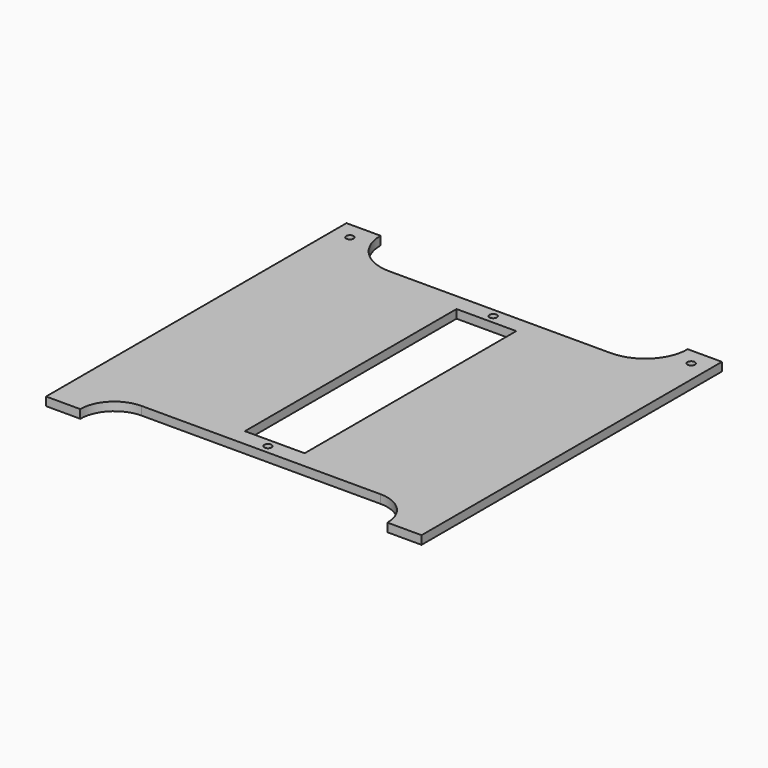
from build123d import *

# Parameters (mm, degrees)
F1_DEPTH = 5
F2_W     = 35
F2_H     = 155
F3_DEPTH = 5.001
F4_R     = 2.15
F5_DEPTH = 5.001


# Not quite as in the source:
# - a feature names something its author has since deleted; it is built from what else it names


with BuildPart() as f1:
    # F0 (on Top) → F1 (new body)
    with BuildSketch(Plane.XY):
        with BuildLine():
            Line((-39.5881515363, 113.7799814343), (-59.5881515363, 113.7799814343))
            Line((-59.5881515363, 113.7799814343), (-59.5881515363, -106.2200185657))
            Line((-59.5881515363, -106.2200185657), (-39.5881515363, -106.2200185657))
            ThreePointArc((-39.5881515363, -106.2200185657), (-33.7302871601, -92.0778829419), (-19.5881515363, -86.2200185657))
            Line((-19.5881515363, -86.2200185657), (120.4118484637, -86.2200185657))
            ThreePointArc((120.4118484637, -86.2200185657), (134.5539840874, -92.0778829419), (140.4118484637, -106.2200185657))
            Line((140.4118484637, -106.2200185657), (160.4118484637, -106.2200185657))
            Line((160.4118484637, -106.2200185657), (160.4118484637, 113.7799814343))
            Line((160.4118484637, 113.7799814343), (140.4118484637, 113.7799814343))
            ThreePointArc((140.4118484637, 113.7799814343), (133.0895179933, 96.1023119047), (115.4118484637, 88.7799814343))
            Line((115.4118484637, 88.7799814343), (-14.5881515363, 88.7799814343))
            ThreePointArc((-14.5881515363, 88.7799814343), (-32.265821066, 96.1023119047), (-39.5881515363, 113.7799814343))
        make_face()
    extrude(amount=F1_DEPTH)

    # F2 (on face) → F3 (cut, through all)
    with BuildSketch(Plane.XY.offset(5)):
        with Locations((50.4118484637, 1.2799814343)):
            Rectangle(F2_W, F2_H)
    extrude(amount=-F3_DEPTH, mode=Mode.SUBTRACT)

    # F4 (on face) → F5 (cut, through all)
    with BuildSketch(Plane.XY.offset(5)):
        with Locations((-49.5881515363, 103.7799814343)):
            Circle(F4_R)
        with Locations((150.4118484637, 103.7799814343)):
            Circle(F4_R)
        with Locations((50.4118484637, 83.7799814343)):
            Circle(F4_R)
        with Locations((50.4118484637, -81.2200185657)):
            Circle(F4_R)
    extrude(amount=-F5_DEPTH, mode=Mode.SUBTRACT)


solid = f1.part
